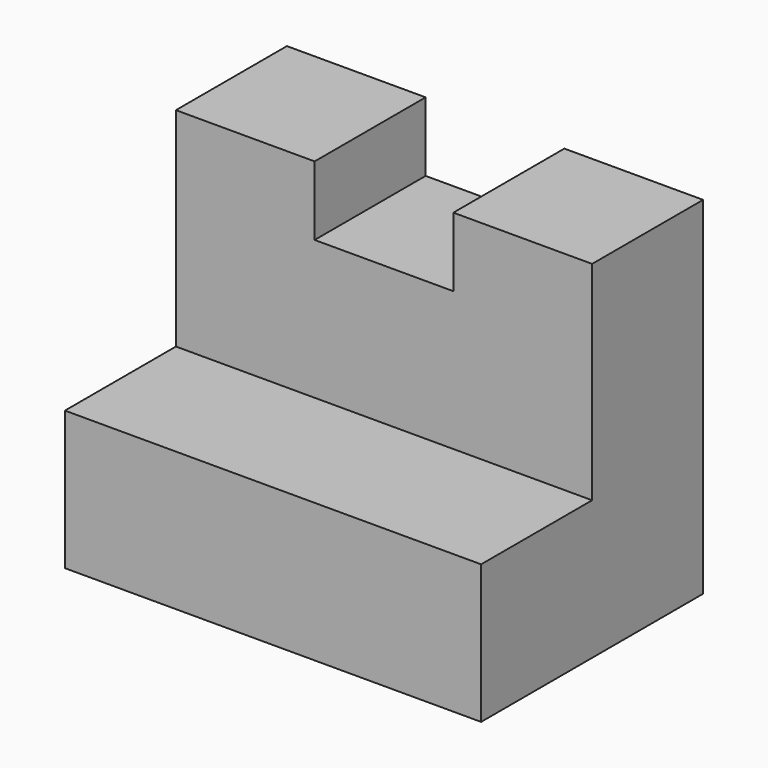
from build123d import *

# Parameters (mm, degrees)
F1_DEPTH = 38.1
F2_W     = 12.7
F2_H     = 6.35
F3_DEPTH = 81
F4_W     = 12.7
F4_H     = 6.35
F5_DEPTH = 81
F6_W     = 12.7
F6_H     = 6.35
F7_DEPTH = 81
F8_DEPTH = 25.401


# Not quite as in the source:
# - an extrude ends at something that could not be found from the text; its depth is read off the source's solid


with BuildPart() as f1:
    # F0 (on Right) → F1 (new body)
    with BuildSketch(Plane.YZ):
        Polygon((0, 0), (0, 31.75), (-12.7, 31.75), (-12.7, 12.7), (-25.4, 12.7), (-25.4, 0), align=None)
    extrude(amount=F1_DEPTH)

    # F2 (on Front) → F3 (cut, through all)
    with BuildSketch(Plane.XZ):
        with Locations((19.05, 29.0438578556)):
            Rectangle(F2_W, F2_H)
    extrude(amount=-F3_DEPTH, mode=Mode.SUBTRACT)

    # F4 (on Front) → F5 (cut, through all)
    with BuildSketch(Plane.XZ):
        with Locations((19.05, 28.5938853313)):
            Rectangle(F4_W, F4_H)
    extrude(amount=-F5_DEPTH, mode=Mode.SUBTRACT)

    # F6 (on Front) → F7 (cut, through all)
    with BuildSketch(Plane.XZ):
        with Locations((19.05, 28.9610116338)):
            Rectangle(F6_W, F6_H)
    extrude(amount=-F7_DEPTH, mode=Mode.SUBTRACT)

    # F4 (on Front) → F8 (cut, through all)
    with BuildSketch(Plane.XZ):
        with Locations((19.05, 28.5938853313)):
            Rectangle(F4_W, F4_H)
    extrude(amount=F8_DEPTH, mode=Mode.SUBTRACT)


solid = f1.part
